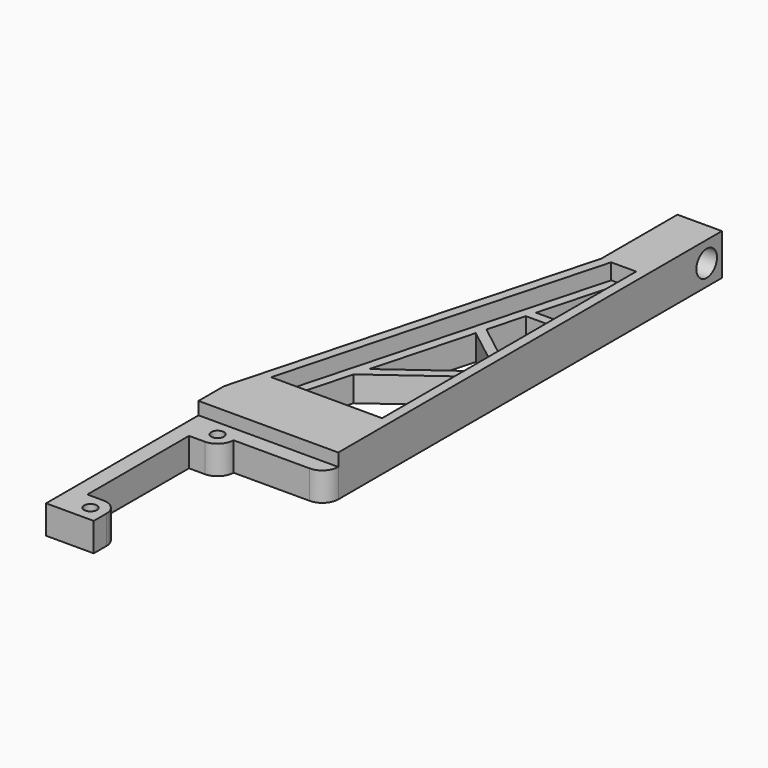
from build123d import *

# Parameters (mm, degrees)
F1_DEPTH  = 13
F0_R      = 2
F2_DEPTH  = 9
F4_DEPTH  = 5
F6_DEPTH  = 8.001
F7_R      = 5
F8_R      = 4.99999
F9_R      = 5
F10_R     = 4.05
F11_DEPTH = 14.001


# Not quite as in the source:
# - a fillet or chamfer is up to 0.001 mm smaller than in the source, because OpenCascade refuses the exact size


with BuildPart() as f1:
    # F0 (on Top) → F1 (new body)
    with BuildSketch(Plane.XY):
        Polygon((-22.5616768954, -33.6060966955), (21.4383231046, -33.6060966955), (21.4383231046, 117.3939033045), (7.4383231046, 117.3939033045), (7.4383231046, 87.3939033045), (-22.5616768954, -23.6060966955), align=None)
    extrude(amount=F1_DEPTH)

    # F0 (on Top) → F2 (join)
    with BuildSketch(Plane.XY):
        Polygon((-17.5616768954, -43.6060966955), (-7.5616768954, -43.6060966955), (-7.5616768954, -38.6060966955), (21.4383231046, -38.6060966955), (21.4383231046, -33.6060966955), (-22.5616768954, -33.6060966955), (-22.5616768954, -93.6060966955), (-7.5616768954, -93.6060966955), (-7.5616768954, -83.6060966955), (-17.5616768954, -83.6060966955), align=None)
        with Locations((-12.5616768954, -88.6060966955)):
            Circle(F0_R, mode=Mode.SUBTRACT)
        with Locations((-12.5616768954, -38.6060966955)):
            Circle(F0_R, mode=Mode.SUBTRACT)
    extrude(amount=F2_DEPTH)

    # F3 (on face) → F4 (cut)
    with BuildSketch(Plane.XY.offset(13)):
        Polygon((-16.4810658851, -12.6060966955), (18.4383231046, -12.6060966955), (18.4383231046, 87.3939033045), (10.545961142, 87.3939033045), align=None)
    extrude(amount=-F4_DEPTH, mode=Mode.SUBTRACT)

    # F5 (on face) → F6 (cut, through all)
    with BuildSketch(Plane.XY.offset(8)):
        Polygon((15.4383231046, 62.3939033045), (15.4383231046, 84.3939033045), (12.8427883685, 84.3939033045), (6.8968424225, 62.3939033045), align=None)
        Polygon((15.4383231046, 38.1328739976), (15.4383231046, 59.3939033045), (6.0860316117, 59.3939033045), (2.95512331, 47.8095425882), align=None)
        Polygon((15.4383231046, 29.3370774792), (15.4383231046, 34.3370774792), (2.1069338573, 44.6712416135), (-6.3520655178, 13.3729439254), align=None)
        Polygon((15.4383231046, -9.6060966955), (15.4383231046, 25.6181227456), (-7.6053455592, 8.7358077721), (-12.562617037, -9.6060966955), align=None)
    extrude(amount=-F6_DEPTH, mode=Mode.SUBTRACT)

    # F7
    f7_edges = [f1.edges().sort_by_distance(p)[0] for p in [
        (21.438323, -38.606097, 4.5),
    ]]
    fillet(f7_edges, radius=F7_R)

    # F8 (radius 5 in the source; OpenCascade refuses exactly that, so slightly less here)
    f8_edges = [f1.edges().sort_by_distance(p)[0] for p in [
        (-7.561677, -43.606097, 4.5),
    ]]
    fillet(f8_edges, radius=F8_R)

    # F9
    f9_edges = [f1.edges().sort_by_distance(p)[0] for p in [
        (-7.561677, -83.606097, 4.5),
    ]]
    fillet(f9_edges, radius=F9_R)

    # F10 (on face) → F11 (cut, through all)
    with BuildSketch(Plane(origin=(7.4383231046, 0, 0), x_dir=(0, -1, 0), z_dir=(-1, 0, 0))):
        with Locations((-111.3939033045, 6.5)):
            Circle(F10_R)
    extrude(amount=-F11_DEPTH, mode=Mode.SUBTRACT)


solid = f1.part
